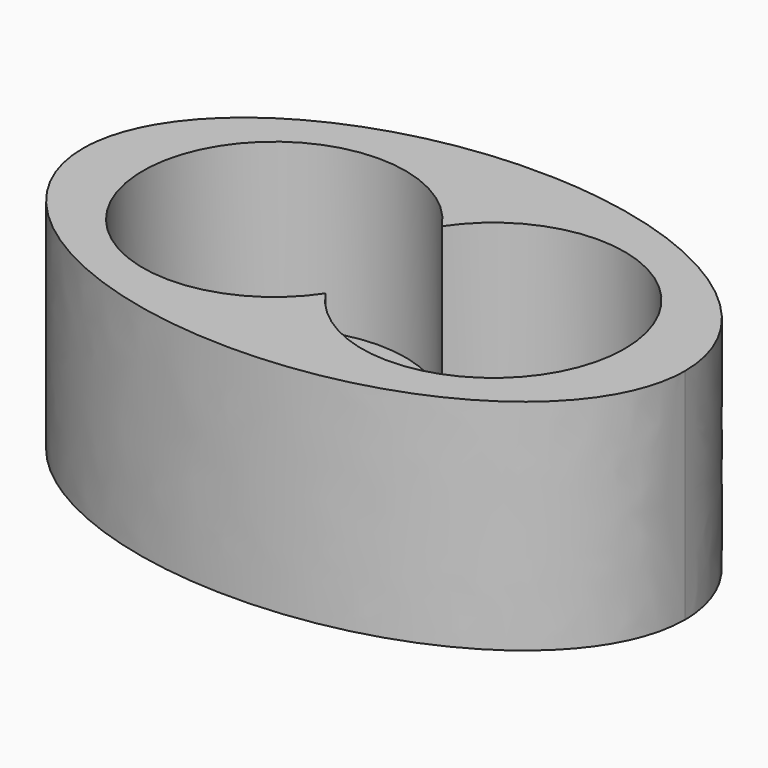
from build123d import *

# Parameters (mm, degrees)
F0_W     = 55
F0_H     = 35
F1_DEPTH = 20
F2_R     = 1
F3_DEPTH = 15
F4_R     = 1
F5_DEPTH = 25


# Not quite as in the source:
# - a feature of the source that left no trace in its solid (it failed there, or was rolled back) is left out
# - a pattern or mirror of a feature is missing from the dataset's text; its kind, count and spacing are read off the source's solid


with BuildPart() as f1:
    # F0 (on Top) → F1 (new body)
    with BuildSketch(Plane.XY):
        with Locations((27.5, 17.5)):
            Rectangle(F0_W, F0_H)
    extrude(amount=F1_DEPTH)

    # F2 (on face) → F3 (cut)
    with BuildSketch(Plane.XY.offset(20)):
        with BuildLine():
            ThreePointArc((27.5, 10.8667504193), (28.9891252931, 14.0358983849), (29.5, 17.5))
            ThreePointArc((29.5, 17.5), (28.9891252931, 20.9641016151), (27.5, 24.1332495807))
            ThreePointArc((27.5, 24.1332495807), (25.5, 17.5), (27.5, 10.8667504193))
        make_face()
        with BuildLine():
            ThreePointArc((27.5, 24.1332495807), (28.9891252931, 20.9641016151), (29.5, 17.5))
            ThreePointArc((29.5, 17.5), (28.9891252931, 14.0358983849), (27.5, 10.8667504193))
            ThreePointArc((27.5, 10.8667504193), (40.9641016151, 6.0108747069), (49.5, 17.5))
            ThreePointArc((49.5, 17.5), (40.9641016151, 28.9891252931), (27.5, 24.1332495807))
        make_face()
        with Locations((37.5, 17.5)):
            Circle(F2_R, mode=Mode.SUBTRACT)
        with BuildLine():
            ThreePointArc((27.5, 10.8667504193), (25.5, 17.5), (27.5, 24.1332495807))
            ThreePointArc((27.5, 24.1332495807), (5.5, 17.5), (27.5, 10.8667504193))
        make_face()
        with Locations((17.5, 17.5)):
            Circle(F2_R, mode=Mode.SUBTRACT)
        with Locations((37.5, 17.5)):
            Circle(F2_R)
    extrude(amount=-F3_DEPTH, mode=Mode.SUBTRACT)

    # F4 (on face) → F5 (cut)
    with BuildSketch(Plane.XY.offset(20)):
        with BuildLine():
            Line((55, 0), (55, 17.5314601511))
            add(Edge.make_bspline(
                [(0, 17.5314601511), (0, 0.0314601511), (27.5, 0.0314601511), (55, 0.0314601511), (55, 17.5314601511)],
                knots=[3.1415926536, 3.1415926536, 3.1415926536, 4.7123889804, 4.7123889804, 6.2831853072, 6.2831853072, 6.2831853072], degree=2, weights=[1, 0.7071067812, 1, 0.7071067812, 1]))
            Line((0, 17.5314601511), (0, 0))
            Line((0, 0), (55, 0))
        make_face()
        with BuildLine():
            add(Edge.make_bspline(
                [(55, 17.5314601511), (55, 34.0122240667), (29.1482147493, 35)],
                knots=[0, 0, 0, 1.5108253036, 1.5108253036, 1.5108253036], degree=2, weights=[1, 0.7279886956, 1]))
            Line((55, 17.5314601511), (55, 35))
            Line((55, 35), (29.1482147493, 35))
        make_face()
        with BuildLine():
            Line((0, 35), (0, 17.5314601511))
            add(Edge.make_bspline(
                [(25.8517852507, 35), (0, 34.0122240667), (0, 17.5314601511)],
                knots=[1.63076735, 1.63076735, 1.63076735, 3.1415926536, 3.1415926536, 3.1415926536], degree=2, weights=[1, 0.7279886956, 1]))
            Line((25.8517852507, 35), (0, 35))
        make_face()
        with Locations((17.5, 17.5)):
            Circle(F4_R)
    f5 = extrude(amount=-F5_DEPTH, mode=Mode.SUBTRACT)

    # F5_copies: F5 across plane
    add(f5.mirror(Plane(origin=(27.5, 0, 0), x_dir=(0, 0, 1), z_dir=(1, 0, 0))), mode=Mode.SUBTRACT)


solid = f1.part
